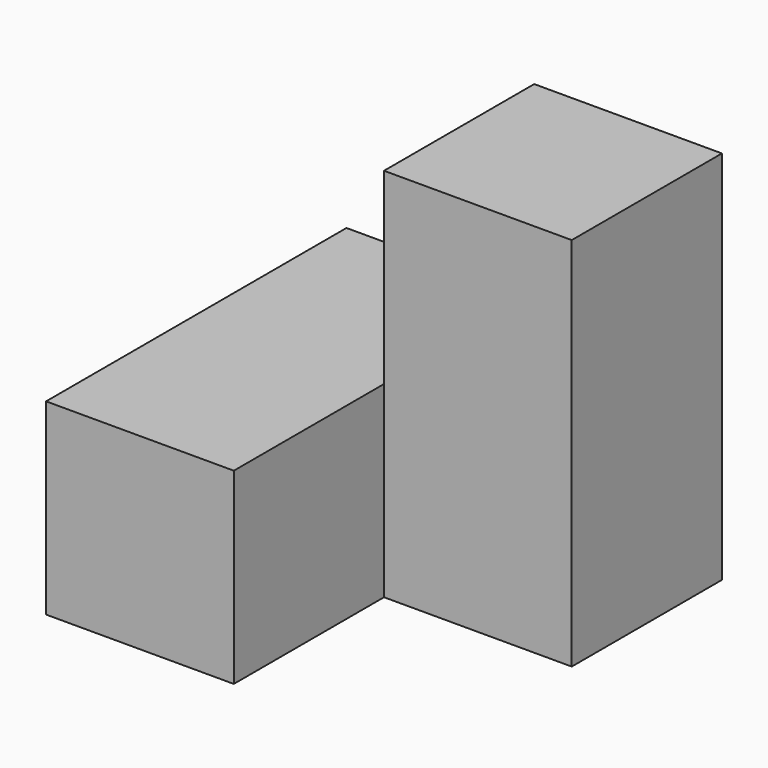
from build123d import *

# Parameters (mm, degrees)
F1_W     = 50.8
F1_H     = 50.8
F2_DEPTH = 25.4
F3_W     = 25.4
F3_H     = 25.4
F4_DEPTH = 25.4
F5_W     = 25.4
F5_H     = 25.4
F6_DEPTH = 25.4


# Not quite as in the source:
# - a variable given as a bare number and used for a length is read in inches; the dataset says mm whatever the document's units were


with BuildPart() as f2:
    # F1 (on Top) → F2 (new body)
    with BuildSketch(Plane.XY):
        Rectangle(F1_W, F1_H)
    extrude(amount=F2_DEPTH)

    # F3 (on face) → F4 (cut)
    with BuildSketch(Plane.XY.offset(25.4)):
        with Locations((12.7, -12.7)):
            Rectangle(F3_W, F3_H)
    extrude(amount=-F4_DEPTH, mode=Mode.SUBTRACT)

    # F5 (on face) → F6 (join)
    with BuildSketch(Plane.XY.offset(25.4)):
        with Locations((12.7, 12.7)):
            Rectangle(F5_W, F5_H)
    extrude(amount=F6_DEPTH)


solid = f2.part
